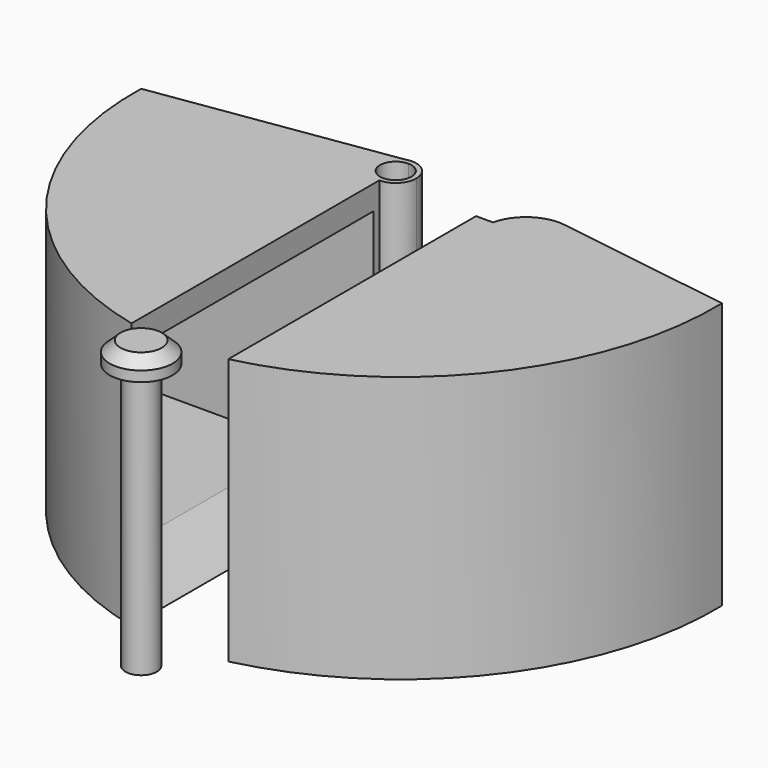
from build123d import *

# Parameters (mm, degrees)
F2_DEPTH      = 55
F3_START      = 2.5
F3_DEPTH      = 47.5
F4_SIZE2      = 14.99999
F4_SIZE       = 2.49999
F4_2_SIZE2    = 14.99999
F4_2_SIZE     = 2.49999
F7_DEPTH      = 55
F8_W          = 8.5
F8_H          = 18.3333333333
F9_DEPTH      = 13.5
F10_DEPTH     = 13.5
F13_T1_DEPTH  = 42.4854968764
F13_T3_DEPTH  = 42.4854968764
F13_T8_DEPTH  = 66.6376604194
F13_T13_DEPTH = 66.6376604194
F14_T1_DEPTH  = 18.3333333333


# Not quite as in the source:
# - a fillet or chamfer that OpenCascade refuses, or shapes differently, is made with other operations: its cross-section is extruded or revolved along the edge and cut away or added
# - two fillets or chamfers of one size are made in one step
# - a fillet or chamfer is up to 0.001 mm smaller than in the source, because OpenCascade refuses the exact size


with BuildPart() as f2:
    # F0 (on Top) → F2 (new body)
    with BuildSketch(Plane.XY):
        with BuildLine():
            ThreePointArc((-60, 75), (-46.5440908417, 33.6199301218), (-10, 10))
            Line((-10, 10), (-10, 75))
            Line((-10, 75), (-60, 75))
        make_face()
    extrude(amount=F2_DEPTH)


with BuildPart() as f2b:
    # F0 (on Top) → F2, piece 2 (new body)
    with BuildSketch(Plane.XY):
        with BuildLine():
            ThreePointArc((10, 10), (46.5440908417, 33.6199301218), (60, 75))
            Line((60, 75), (10, 75))
            Line((10, 75), (10, 10))
        make_face()
    extrude(amount=F2_DEPTH)


with BuildPart() as f3_tool:
    # F1 (on Top) → F3 (new body)
    with BuildSketch(Plane.XY.offset(F3_START)):
        with BuildLine():
            Line((-9, 72.5), (-56, 72.5))
            ThreePointArc((-56, 72.5), (-42.2168279916, 34.8884847399), (-9, 12.5))
            Line((-9, 12.5), (-9, 72.5))
        make_face()
        with BuildLine():
            ThreePointArc((9, 12.5), (42.2168279916, 34.8884847399), (56, 72.5))
            Line((56, 72.5), (9, 72.5))
            Line((9, 72.5), (9, 12.5))
        make_face()
    extrude(amount=F3_DEPTH)


with BuildPart() as f2_1:
    add(f2.part)

    # F3: cut by f3_tool
    add(f3_tool.part, mode=Mode.SUBTRACT)

    # F4#2 (size 2.5 and 15 in the source; OpenCascade refuses exactly that, so slightly less here)
    f4_2_edges = [f2_1.edges().sort_by_distance(p)[0] for p in [
        (-10, 42.648042, 2.5),
    ]]
    chamfer(f4_2_edges, length=F4_2_SIZE, length2=F4_2_SIZE2)

    # F6 (on Top) → F7 (join, through all)
    with BuildSketch(Plane.XY):
        with BuildLine():
            ThreePointArc((-12.7386127875, 75), (-8.2078789587, 74.3963261459), (-5.75, 78.25))
            ThreePointArc((-5.75, 78.25), (-6.99479618, 81.25520382), (-10, 82.5))
            Line((-10, 82.5), (-10, 81.5))
            ThreePointArc((-10, 81.5), (-7.7019029611, 80.5480970389), (-6.75, 78.25))
            ThreePointArc((-6.75, 78.25), (-7.7019029611, 75.9519029611), (-10, 75))
            Line((-10, 75), (-12.7386127875, 75))
        make_face()
        with BuildLine():
            Line((-11.2469437653, 82.3129584352), (-10, 82.5))
            ThreePointArc((-10, 82.5), (-10.630446925, 82.4529794997), (-11.2469437653, 82.3129584352))
        make_face()
        with BuildLine():
            Line((-10, 81.5), (-10, 82.5))
            Line((-10, 82.5), (-11.2469437653, 82.3129584352))
            ThreePointArc((-11.2469437653, 82.3129584352), (-14.1642532977, 79.0994083072), (-12.7386127875, 75))
            Line((-12.7386127875, 75), (-10, 75))
            ThreePointArc((-10, 75), (-13.25, 78.25), (-10, 81.5))
        make_face()
        with BuildLine():
            Line((-60, 75), (-12.7386127875, 75))
            ThreePointArc((-12.7386127875, 75), (-14.1642532977, 79.0994083072), (-11.2469437653, 82.3129584352))
            Line((-11.2469437653, 82.3129584352), (-60, 75))
        make_face()
    extrude(amount=F7_DEPTH)

    # F8 (on Right) → F10 (cut)
    with BuildSketch(Plane.YZ):
        with Locations((78.25, 27.5)):
            Rectangle(F8_W, F8_H)
    extrude(amount=-F10_DEPTH, mode=Mode.SUBTRACT)

    # F14: fillet of radius 8.5 on 1 edges, made by hand

    # F14_s2 → F14_t1 (cut)
    with BuildSketch(Plane.XY.offset(18.3333333333)):
        with BuildLine():
            ThreePointArc((-23.0539810113, 80.5419028483), (-16.9907899078, 79.1493553646), (-13.5, 74))
            Line((-13.5, 74), (-13.5, 81.975))
            Line((-13.5, 81.975), (-23.0539810113, 80.5419028483))
        make_face()
    extrude(amount=F14_T1_DEPTH, mode=Mode.SUBTRACT)


with BuildPart() as f2b_1:
    add(f2b.part)

    # F3: cut by f3_tool
    add(f3_tool.part, mode=Mode.SUBTRACT)

    # F4 (size 2.5 and 15 in the source; OpenCascade refuses exactly that, so slightly less here)
    f4_edges = [f2b_1.edges().sort_by_distance(p)[0] for p in [
        (10, 42.648042, 2.5),
    ]]
    chamfer(f4_edges, length=F4_SIZE, length2=F4_SIZE2)

    # F6 (on Top) → F7, piece 2 (join, through all)
    with BuildSketch(Plane.XY):
        with BuildLine():
            ThreePointArc((12.7386127875, 75), (13.8536738541, 76.4578789587), (14.25, 78.25))
            ThreePointArc((14.25, 78.25), (13.4177486012, 80.7761620096), (11.2469437653, 82.3129584352))
            Line((11.2469437653, 82.3129584352), (10, 82.5))
            Line((10, 82.5), (10, 81.5))
            ThreePointArc((10, 81.5), (12.2980970389, 80.5480970389), (13.25, 78.25))
            ThreePointArc((13.25, 78.25), (12.2980970389, 75.9519029611), (10, 75))
            Line((10, 75), (12.7386127875, 75))
        make_face()
        with BuildLine():
            ThreePointArc((11.2469437653, 82.3129584352), (13.4177486012, 80.7761620096), (14.25, 78.25))
            ThreePointArc((14.25, 78.25), (13.8536738541, 76.4578789587), (12.7386127875, 75))
            Line((12.7386127875, 75), (60, 75))
            Line((60, 75), (11.2469437653, 82.3129584352))
        make_face()
        with BuildLine():
            Line((10, 82.5), (11.2469437653, 82.3129584352))
            ThreePointArc((11.2469437653, 82.3129584352), (10.630446925, 82.4529794997), (10, 82.5))
        make_face()
        with BuildLine():
            ThreePointArc((10, 82.5), (6.0078201443, 76.7922620263), (12.7386127875, 75))
            Line((12.7386127875, 75), (10, 75))
            ThreePointArc((10, 75), (6.75, 78.25), (10, 81.5))
            Line((10, 81.5), (10, 82.5))
        make_face()
    extrude(amount=F7_DEPTH)

    # F8 (on Right) → F9 (cut)
    with BuildSketch(Plane.YZ):
        with Locations((78.25, 45.8333333333)):
            Rectangle(F8_W, F8_H)
        with Locations((78.25, 9.1666666667)):
            Rectangle(F8_W, F8_H)
    extrude(amount=F9_DEPTH, mode=Mode.SUBTRACT)

    # F13: fillet of radius 8.5 on 2 edges, made by hand

    # F13_s2 → F13_t1 (cut)
    with BuildSketch(Plane.XY.offset(36.6666666667)):
        with BuildLine():
            ThreePointArc((23.0539810113, 80.5419028483), (16.9907899078, 79.1493553646), (13.5, 74))
            Line((13.5, 74), (13.5, 81.975))
            Line((13.5, 81.975), (23.0539810113, 80.5419028483))
        make_face()
    extrude(amount=F13_T1_DEPTH, mode=Mode.SUBTRACT)

    # F13_s4 → F13_t3 (cut)
    with BuildSketch(Plane.XY.offset(-24.152163543)):
        with BuildLine():
            ThreePointArc((23.0539810113, 80.5419028483), (16.9907899078, 79.1493553646), (13.5, 74))
            Line((13.5, 74), (13.5, 81.975))
            Line((13.5, 81.975), (23.0539810113, 80.5419028483))
        make_face()
    extrude(amount=F13_T3_DEPTH, mode=Mode.SUBTRACT)


with BuildPart() as f12:
    # F11 (on Front) → F12 (revolve)
    with BuildSketch(Plane.XZ):
        Polygon((-3.25, 0), (0, 0), (0, 59.25), (-4.25, 59.25), (-6.5, 57.125), (-6.5, 55), (-3.25, 55), align=None)
    revolve(axis=Axis((0, 0, 29.625), (0, 0, 1)))


with BuildPart() as f13_tool6:
    # F13_s7 → F13_t8 (new body)
    with BuildSketch(Plane.XY.offset(12.5145031236)):
        with BuildLine():
            ThreePointArc((23.0539810113, 80.5419028483), (16.9907899078, 79.1493553646), (13.5, 74))
            Line((13.5, 74), (13.5, 81.975))
            Line((13.5, 81.975), (23.0539810113, 80.5419028483))
        make_face()
    extrude(amount=F13_T8_DEPTH)

    split(bisect_by=Plane.XY.offset(18.3333333333), keep=Keep.BOTTOM)


with BuildPart() as f2b_2:
    add(f2b_1.part)

    # F13_t5: cut F13_tool6
    add(f13_tool6.part, mode=Mode.SUBTRACT)


with BuildPart() as f13_tool11:
    # F13_s12 → F13_t13 (new body)
    with BuildSketch(Plane.XY.offset(-24.152163543)):
        with BuildLine():
            ThreePointArc((23.0539810113, 80.5419028483), (16.9907899078, 79.1493553646), (13.5, 74))
            Line((13.5, 74), (13.5, 81.975))
            Line((13.5, 81.975), (23.0539810113, 80.5419028483))
        make_face()
    extrude(amount=F13_T13_DEPTH)

    split(bisect_by=Plane.XY.offset(36.6666666667), keep=Keep.TOP)


with BuildPart() as f2b_3:
    add(f2b_2.part)

    # F13_t10: cut F13_tool11
    add(f13_tool11.part, mode=Mode.SUBTRACT)


solid = Compound([f2_1.part, f12.part, f2b_3.part])
